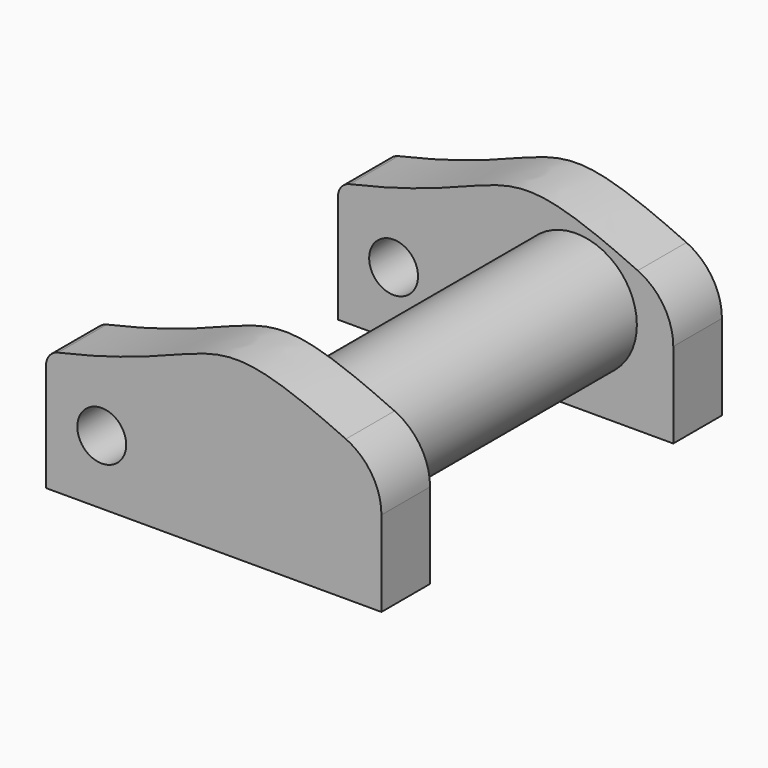
from build123d import *

# Parameters (mm, degrees)
F1_DEPTH = 25.4
F2_R     = 25.4
F3_DEPTH = 127
F6_R     = 25.3967781552
F7_R     = 10.211273354
F8_DEPTH = 211.42987


# Not quite as in the source:
# - a feature of the source that left no trace in its solid (it failed there, or was rolled back) is left out
# - a pattern or mirror of a feature is missing from the dataset's text; its kind, count and spacing are read off the source's solid


with BuildPart() as f1:
    # F0 (on Front) → F1 (new body)
    with BuildSketch(Plane.XZ):
        with BuildLine():
            Line((-140.086213054, 0), (0, 0))
            Line((0, 0), (0, 51.7864115536))
            add(Edge.make_bspline(
                [(-135.121182604, 51.4369904306), (-57.8541277154, 68.705081156), (-79.1493766813, 89.948796737), (0, 51.7864115536)],
                knots=[0.0132853618, 0.0132853618, 0.0132853618, 0.0132853618, 0.6502691411, 0.6502691411, 0.6502691411, 0.6502691411], degree=3))
            ThreePointArc((-135.121182604, 51.4369904306), (-138.6918692488, 49.210252186), (-140.086213054, 45.2398653435))
            Line((-140.086213054, 45.2398653435), (-140.086213054, 0))
        make_face()
    extrude(amount=F1_DEPTH)


with BuildPart() as f1_copies_1:
    # F1_copies: instance of F1
    add(f1.part.mirror(Plane(origin=(0, -88.9, 1e-06), x_dir=(0, 0, -1), z_dir=(0, -1, 0))))


with BuildPart() as f1_1:
    add(f1.part)

    add(f1_copies_1.part)  # F3 merges F1_copies_1
    # F2 (on face) → F3 (join)
    with BuildSketch(Plane.XZ.offset(25.4)):
        with Locations((-40.6125485897, 38.6877208911)):
            Circle(F2_R)
    extrude(amount=F3_DEPTH)

    # F6
    f6_edges = [f1_1.edges().sort_by_distance(p)[0] for p in [
        (0, -12.7, 51.786412),
        (0, -165.1, 51.786412),
    ]]
    fillet(f6_edges, radius=F6_R)

    # F7 (on face) → F8 (cut)
    with BuildSketch(Plane(origin=(0, 0, 0), x_dir=(-1, 0, 0), z_dir=(0, 1, 0))):
        with Locations((116.8357878923, 26.8229749054)):
            Circle(F7_R)
    extrude(amount=-F8_DEPTH, mode=Mode.SUBTRACT)


solid = f1_1.part
